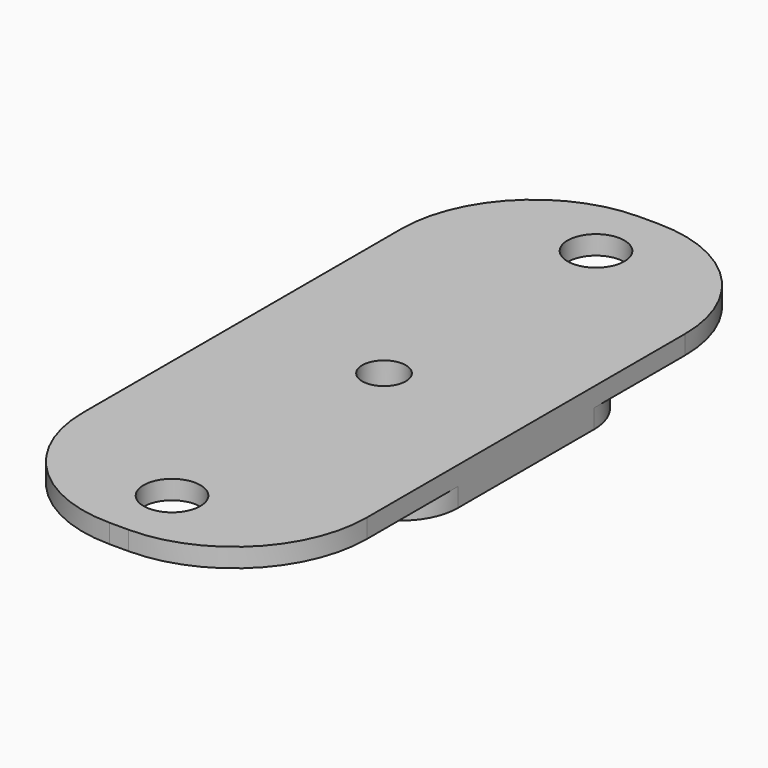
from build123d import *

# Parameters (mm, degrees)
F0_R     = 2.5
F0_R_2   = 1.15
F1_DEPTH = 1
F2_W     = 15
F2_H     = 15
F2_R     = 5
F2_R_2   = 2.5
F2_R_3   = 1.15
F3_DEPTH = 1
F4_R     = 3
F6_W     = 15
F6_H     = 35
F6_R     = 1.5
F6_R_2   = 1.15
F7_DEPTH = 1
F8_R     = 7


# Not quite as in the source:
# - a feature of the source that left no trace in its solid (it failed there, or was rolled back) is left out


with BuildPart() as f1:
    # F0 (on Top) → F1 (new body)
    with BuildSketch(Plane.XY):
        Circle(F0_R)
        Circle(F0_R_2, mode=Mode.SUBTRACT)
    extrude(amount=F1_DEPTH)

    # F2 (on face) → F3 (join)
    with BuildSketch(Plane(origin=(0, 0, 0), x_dir=(1, 0, 0), z_dir=(0, 0, -1))):
        Rectangle(F2_W, F2_H)
        Circle(F2_R, mode=Mode.SUBTRACT)
        Circle(F2_R)
        Circle(F2_R_2, mode=Mode.SUBTRACT)
        Circle(F2_R_2)
        Circle(F2_R_3, mode=Mode.SUBTRACT)
    extrude(amount=F3_DEPTH)

    # F4
    f4_edges = [f1.edges().sort_by_distance(p)[0] for p in [
        (-7.5, 7.5, -0.5),
        (7.5, 7.5, -0.5),
        (-7.5, -7.5, -0.5),
        (7.5, -7.5, -0.5),
    ]]
    fillet(f4_edges, radius=F4_R)

    # F6 (on face) → F7 (join)
    with BuildSketch(Plane.XY):
        Rectangle(F6_W, F6_H)
        with Locations((0, -14)):
            Circle(F6_R, mode=Mode.SUBTRACT)
        Circle(F6_R_2, mode=Mode.SUBTRACT)
        with Locations((0, 14)):
            Circle(F6_R, mode=Mode.SUBTRACT)
    extrude(amount=F7_DEPTH)

    # F8
    f8_edges = [f1.edges().sort_by_distance(p)[0] for p in [
        (-7.5, 17.5, 0.5),
        (7.5, 17.5, 0.5),
        (7.5, -17.5, 0.5),
        (-7.5, -17.5, 0.5),
    ]]
    fillet(f8_edges, radius=F8_R)


solid = f1.part
